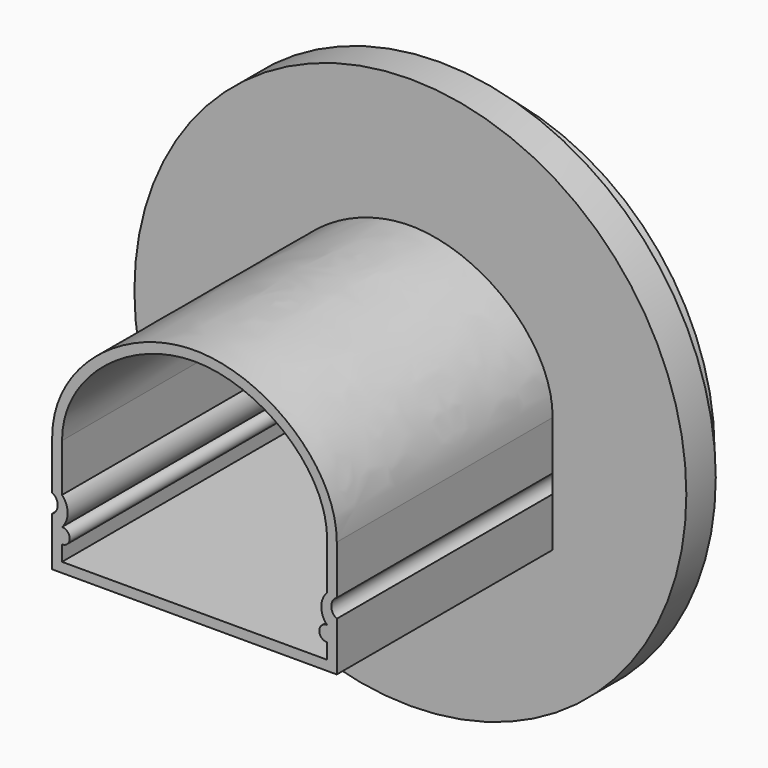
from build123d import *

# Parameters (mm, degrees)
F1_DEPTH = 25
F2_R     = 22.5
F2_R_2   = 20
F2_R_3   = 0.5
F3_DEPTH = 3
F5_DEPTH = 3


# Not quite as in the source:
# - the dataset's text gives a spline's control points without its knots; the knots are read off the source's solid
# - a feature names something its author has since deleted; it is built from what else it names


with BuildPart() as f1:
    # F0 (on Front) → F1 (new body)
    with BuildSketch(Plane.XZ):
        with BuildLine():
            Line((-11.6, 4), (-11.6, 0))
            Line((-11.6, 0), (11.6, 0))
            Line((11.6, 0), (11.6, 4))
            ThreePointArc((11.6, 4), (11.15, 4.75), (11.6, 5.5))
            Line((11.6, 5.5), (11.6, 9.5))
            add(Edge.make_bspline(
                [(11.6, 9.5), (11.6, 14.9057612107), (5.7087616122, 19.5), (0, 19.5)],
                knots=[0, 0, 0, 0, 15.3153517753, 15.3153517753, 15.3153517753, 15.3153517753], degree=3))
            add(Edge.make_bspline(
                [(-11.6, 9.5), (-11.6, 14.9057612107), (-5.7087616122, 19.5), (0, 19.5)],
                knots=[0, 0, 0, 0, 15.3153517753, 15.3153517753, 15.3153517753, 15.3153517753], degree=3))
            Line((-11.6, 9.5), (-11.6, 5.5))
            ThreePointArc((-11.6, 5.5), (-11.15, 4.75), (-11.6, 4))
        make_face()
        with BuildLine():
            Line((10.8, 0.8), (0, 0.8))
            Line((0, 0.8), (-10.8, 0.8))
            Line((-10.8, 0.8), (-10.8, 2.05))
            ThreePointArc((-10.8, 2.05), (-10.175, 2.675), (-10.8, 3.3))
            ThreePointArc((-10.8, 3.3), (-10.3379229861, 4.45), (-10.8, 5.6))
            Line((-10.8, 5.6), (-10.8, 9.5))
            add(Edge.make_bspline(
                [(-10.8, 9.5), (-10.8, 10.1030663269), (-10.6361560663, 11.2884100286), (-9.7228728088, 13.5496398504), (-7.603062861, 16.0660942728), (-4.0104787703, 18.1666619497), (-1.3198877666, 18.7), (0, 18.7)],
                knots=[0, 0, 0, 0, 0.125, 0.25, 0.5, 0.75, 1, 1, 1, 1], degree=3))
            add(Edge.make_bspline(
                [(10.8, 9.5), (10.8, 10.1030663269), (10.6361560663, 11.2884100286), (9.7228728088, 13.5496398504), (7.603062861, 16.0660942728), (4.0104787703, 18.1666619497), (1.3198877666, 18.7), (0, 18.7)],
                knots=[0, 0, 0, 0, 0.125, 0.25, 0.5, 0.75, 1, 1, 1, 1], degree=3))
            Line((10.8, 9.5), (10.8, 5.6))
            ThreePointArc((10.8, 5.6), (10.3379229861, 4.45), (10.8, 3.3))
            ThreePointArc((10.8, 3.3), (10.175, 2.675), (10.8, 2.05))
            Line((10.8, 2.05), (10.8, 0.8))
        make_face(mode=Mode.SUBTRACT)
    extrude(amount=F1_DEPTH)


with BuildPart() as f3:
    # F2 (on Front) → F3 (new body)
    with BuildSketch(Plane.XZ):
        with Locations((0, 7.5230388902)):
            Circle(F2_R)
        with Locations((0, 7.5230388902)):
            Circle(F2_R_2, mode=Mode.SUBTRACT)
        with Locations((0, 7.5230388902)):
            Circle(F2_R_2)
        with Locations((0, -7.6888706521)):
            Circle(F2_R_3, mode=Mode.SUBTRACT)
        with BuildLine():
            add(Edge.make_bspline(
                [(0, 19.5), (-5.7087616122, 19.5), (-11.6, 14.9057612107), (-11.6, 9.5)],
                knots=[0, 0, 0, 0, 1, 1, 1, 1], degree=3))
            add(Edge.make_bspline(
                [(11.6, 9.5), (11.6, 14.9057612107), (5.7087616122, 19.5), (0, 19.5)],
                knots=[0, 0, 0, 0, 1, 1, 1, 1], degree=3))
            Line((11.6, 9.5), (11.6, 5.5))
            Line((11.6, 5.5), (11.6, 4))
            Line((11.6, 4), (11.6, 0))
            Line((11.6, 0), (-11.6, 0))
            Line((-11.6, 0), (-11.6, 4))
            Line((-11.6, 4), (-11.6, 5.5))
            Line((-11.6, 5.5), (-11.6, 9.5))
        make_face(mode=Mode.SUBTRACT)
    extrude(amount=F3_DEPTH)


with BuildPart() as f5:
    # F4 (on Front) → F5 (new body)
    with BuildSketch(Plane.XZ):
        with BuildLine():
            Line((-11.6, 9.5), (-11.6, 8.0917893678))
            Line((-11.6, 8.0917893678), (-11.5470053838, 8))
            Line((-11.5470053838, 8), (-11.6, 7.9082106322))
            Line((-11.6, 7.9082106322), (-11.6, 3.9082106322))
            Line((-11.6, 3.9082106322), (-9.8149545762, 7))
            Line((-9.8149545762, 7), (-5.7735026919, 7))
            Line((-5.7735026919, 7), (-3.7527767497, 3.5))
            Line((-3.7527767497, 3.5), (-5.7735026919, 0))
            Line((-5.7735026919, 0), (-3.4641016151, 0))
            Line((-3.4641016151, 0), (-2.0207259422, 2.5))
            Line((-2.0207259422, 2.5), (2.0207259422, 2.5))
            Line((2.0207259422, 2.5), (3.4641016151, 0))
            Line((3.4641016151, 0), (5.7735026919, 0))
            Line((5.7735026919, 0), (3.7527767497, 3.5))
            Line((3.7527767497, 3.5), (5.7735026919, 7))
            Line((5.7735026919, 7), (9.8149545762, 7))
            Line((9.8149545762, 7), (11.6, 3.9082106322))
            Line((11.6, 3.9082106322), (11.6, 7.9082106322))
            Line((11.6, 7.9082106322), (11.5470053838, 8))
            Line((11.5470053838, 8), (11.6, 8.0917893678))
            Line((11.6, 8.0917893678), (11.6, 9.5))
            add(Edge.make_bspline(
                [(11.6, 9.5), (11.6, 10.2119185774), (11.4978229092, 10.9097621854), (11.3073418694, 11.5848906163)],
                knots=[0, 0, 0, 0, 0.1316962681, 0.1316962681, 0.1316962681, 0.1316962681], degree=3))
            Line((11.3073418694, 11.5848906163), (9.8149545762, 9))
            Line((9.8149545762, 9), (5.7735026919, 9))
            Line((5.7735026919, 9), (3.7527767497, 12.5))
            Line((3.7527767497, 12.5), (5.7735026919, 16))
            Line((5.7735026919, 16), (8.5327536542, 16))
            add(Edge.make_bspline(
                [(8.5327536542, 16), (6.9682227077, 17.4875332287), (4.9454375756, 18.606013275), (2.8034534401, 19.1442762052)],
                knots=[0.453411459, 0.453411459, 0.453411459, 0.453411459, 0.8355950075, 0.8355950075, 0.8355950075, 0.8355950075], degree=3))
            Line((2.8034534401, 19.1442762052), (4.0414518843, 17))
            Line((4.0414518843, 17), (2.0207259422, 13.5))
            Line((2.0207259422, 13.5), (-2.0207259422, 13.5))
            Line((-2.0207259422, 13.5), (-4.0414518843, 17))
            Line((-4.0414518843, 17), (-2.8034534401, 19.1442762052))
            add(Edge.make_bspline(
                [(-2.8034534401, 19.1442762052), (-4.9454375756, 18.606013275), (-6.9682227077, 17.4875332287), (-8.5327536542, 16)],
                knots=[0.1644049925, 0.1644049925, 0.1644049925, 0.1644049925, 0.546588541, 0.546588541, 0.546588541, 0.546588541], degree=3))
            Line((-8.5327536542, 16), (-5.7735026919, 16))
            Line((-5.7735026919, 16), (-3.7527767497, 12.5))
            Line((-3.7527767497, 12.5), (-5.7735026919, 9))
            Line((-5.7735026919, 9), (-9.8149545762, 9))
            Line((-9.8149545762, 9), (-11.3073418694, 11.5848906163))
            add(Edge.make_bspline(
                [(-11.3073418694, 11.5848906163), (-11.4978229092, 10.9097621854), (-11.6, 10.2119185774), (-11.6, 9.5)],
                knots=[0.8683037319, 0.8683037319, 0.8683037319, 0.8683037319, 1, 1, 1, 1], degree=3))
        make_face()
        Polygon((-2.0207259422, 11.5), (2.0207259422, 11.5), (4.0414518843, 8), (2.0207259422, 4.5), (-2.0207259422, 4.5), (-4.0414518843, 8), align=None, mode=Mode.SUBTRACT)
    extrude(amount=-F5_DEPTH)



with BuildPart() as f5b:
    # F4 (on Front) → F5, piece 2 (new body)
    with BuildSketch(Plane.XZ):
        Polygon((11.6, 3.0917893678), (9.8149545762, 0), (11.6, 0), align=None)
    extrude(amount=-F5_DEPTH)


with BuildPart() as f5c:
    # F4 (on Front) → F5, piece 3 (new body)
    with BuildSketch(Plane.XZ):
        Polygon((-9.8149545762, 0), (-11.6, 3.0917893678), (-11.6, 0), align=None)
    extrude(amount=-F5_DEPTH)


with BuildPart() as f5_1:
    add(f5.part)

    add(f5b.part)  # F5#4 merges F5b

    add(f5c.part)  # F5#4 merges F5c
    # F2 (on Front) → F5, piece 4 (join)
    with BuildSketch(Plane.XZ):
        with Locations((0, 7.5230388902)):
            Circle(F2_R_2)
        with Locations((0, -7.6888706521)):
            Circle(F2_R_3, mode=Mode.SUBTRACT)
        with BuildLine():
            add(Edge.make_bspline(
                [(0, 19.5), (-5.7087616122, 19.5), (-11.6, 14.9057612107), (-11.6, 9.5)],
                knots=[0, 0, 0, 0, 1, 1, 1, 1], degree=3))
            add(Edge.make_bspline(
                [(11.6, 9.5), (11.6, 14.9057612107), (5.7087616122, 19.5), (0, 19.5)],
                knots=[0, 0, 0, 0, 1, 1, 1, 1], degree=3))
            Line((11.6, 9.5), (11.6, 5.5))
            Line((11.6, 5.5), (11.6, 4))
            Line((11.6, 4), (11.6, 0))
            Line((11.6, 0), (-11.6, 0))
            Line((-11.6, 0), (-11.6, 4))
            Line((-11.6, 4), (-11.6, 5.5))
            Line((-11.6, 5.5), (-11.6, 9.5))
        make_face(mode=Mode.SUBTRACT)
    extrude(amount=-F5_DEPTH)


solid = Compound([f1.part, f3.part, f5_1.part])
